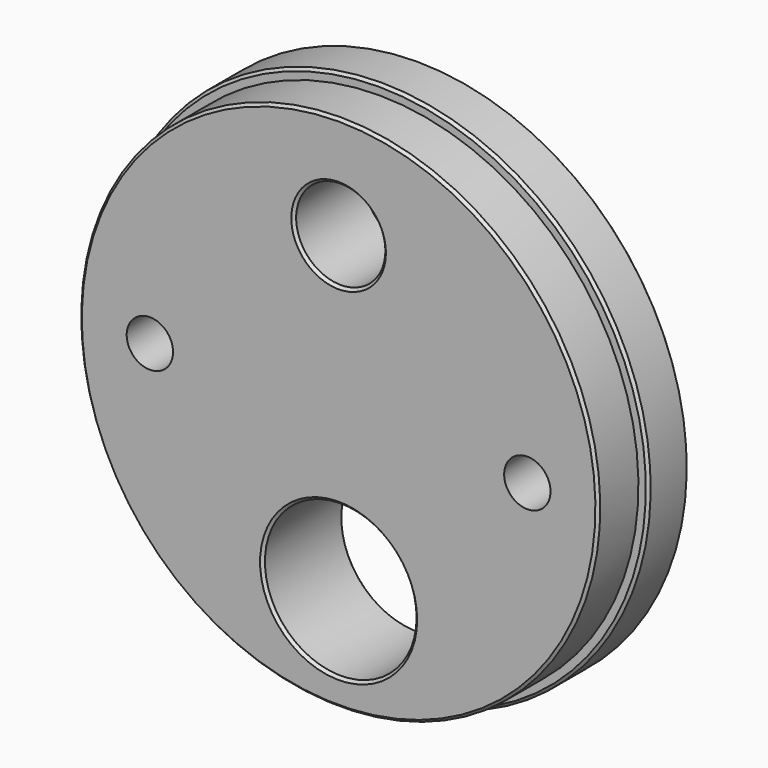
from build123d import *

# Parameters (mm, degrees)
F3_D           = 14.2875
F4_D           = 8.4074
F4_CSINK_D     = 10.922
F4_CSINK_ANGLE = 90
F5_D           = 4.3688
F5_CSINK_D     = 8.128
F5_CSINK_ANGLE = 82
F6_SIZE2       = 0.254
F6_SIZE        = 0.254


with BuildPart() as f1:
    # F0 (on Right) → F1 (revolve)
    with BuildSketch(Plane.YZ):
        Polygon((4.7498, 24.4475), (0, 24.4475), (0, 0), (9.4996, 0), (9.4996, 25.4), (4.7498, 25.4), align=None)
    revolve(axis=Axis((0, 5.1186173223, 0), (0, 1, 0)))

    # F3 (through all)
    with Locations(Plane(origin=(0, 9.4996, 0), x_dir=(-1, 0, 0), z_dir=(0, 1, 0))):
        with Locations((0, -14.732)):
            Hole(F3_D / 2)

    # F4 (through all)
    with Locations(Plane(origin=(0, 9.4996, 0), x_dir=(-1, 0, 0), z_dir=(0, 1, 0))):
        with Locations((0, 14.732)):
            CounterSinkHole(F4_D / 2, F4_CSINK_D / 2, counter_sink_angle=F4_CSINK_ANGLE)

    # F5 (through all)
    with Locations(Plane(origin=(0, 9.4996, 0), x_dir=(-1, 0, 0), z_dir=(0, 1, 0))):
        with Locations((-17.78, 0), (17.78, 0)):
            CounterSinkHole(F5_D / 2, F5_CSINK_D / 2, counter_sink_angle=F5_CSINK_ANGLE)

    # F6
    f6_edges = [f1.edges().sort_by_distance(p)[0] for p in [
        (0, 9.4996, -25.4),
        (0, 0, -24.4475),
        (0, 4.7498, -25.4),
        (7.14375, 0, -14.732),
        (4.2037, 0, 14.732),
        (7.14375, 9.4996, -14.732),
    ]]
    chamfer(f6_edges, length=F6_SIZE, length2=F6_SIZE2)


solid = f1.part
